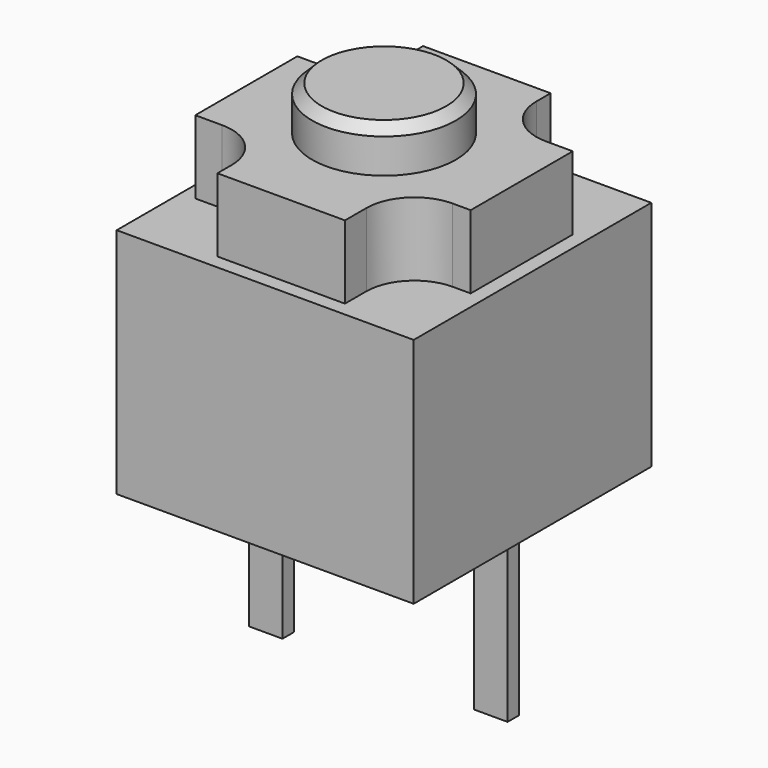
from build123d import *

# Parameters (mm, degrees)
F0_W            = 6.2
F0_H            = 6.2
F1_DEPTH        = 4.85
F3_DEPTH        = 1.53
F3_COPIES_COUNT = 4
F4_R            = 1.5
F5_DEPTH        = 0.92
F6_SIZE         = 0.2
F7_W            = 0.7
F7_H            = 3.5
F8_DEPTH        = 0.15


# Not quite as in the source:
# - a pattern or mirror of a feature is missing from the dataset's text; its kind, count and spacing are read off the source's solid


with BuildPart() as f1:
    # F0 (on Top) → F1 (new body)
    with BuildSketch(Plane.XY):
        Rectangle(F0_W, F0_H)
    extrude(amount=F1_DEPTH)

    # F2 (on face) → F3 (join)
    with BuildSketch(Plane.XY.offset(4.85)):
        with BuildLine():
            Line((1.2382979223, 2.8), (0, 2.8))
            Line((0, 2.8), (0, 0))
            Line((0, 0), (2.8, 0))
            Line((2.8, 0), (2.8, 1.4253550908))
            Line((2.8, 1.4253550908), (2.2382979223, 1.4253550908))
            ThreePointArc((2.2382979223, 1.4253550908), (1.5311911411, 1.7182483096), (1.2382979223, 2.4253550908))
            Line((1.2382979223, 2.4253550908), (1.2382979223, 2.8))
        make_face()
    f3 = extrude(amount=F3_DEPTH)

    # F3_copies: F3 ×4 about axis
    f3_copies_axis = Axis((0, 0, 0), (0, 0, 1))
    for i in range(1, F3_COPIES_COUNT):
        add(f3.rotate(f3_copies_axis, i * 360 / F3_COPIES_COUNT))

    # F4 (on face) → F5 (join)
    with BuildSketch(Plane.XY.offset(6.38)):
        Circle(F4_R)
    extrude(amount=F5_DEPTH)

    # F6
    f6_edges = [f1.edges().sort_by_distance(p)[0] for p in [
        (-1.5, 0, 7.3),
    ]]
    chamfer(f6_edges, length=F6_SIZE)

    # F7 (on Front) → F8 (join, symmetric)
    with BuildSketch(Plane.XZ):
        with Locations((-2.35, -1.75)):
            Rectangle(F7_W, F7_H)
    f8 = extrude(amount=F8_DEPTH, both=True)

    # F8_copies: F8 across plane
    add(f8.mirror(Plane(origin=(0, 0, 0), x_dir=(0, 0, 1), z_dir=(1, 0, 0))))


solid = f1.part
